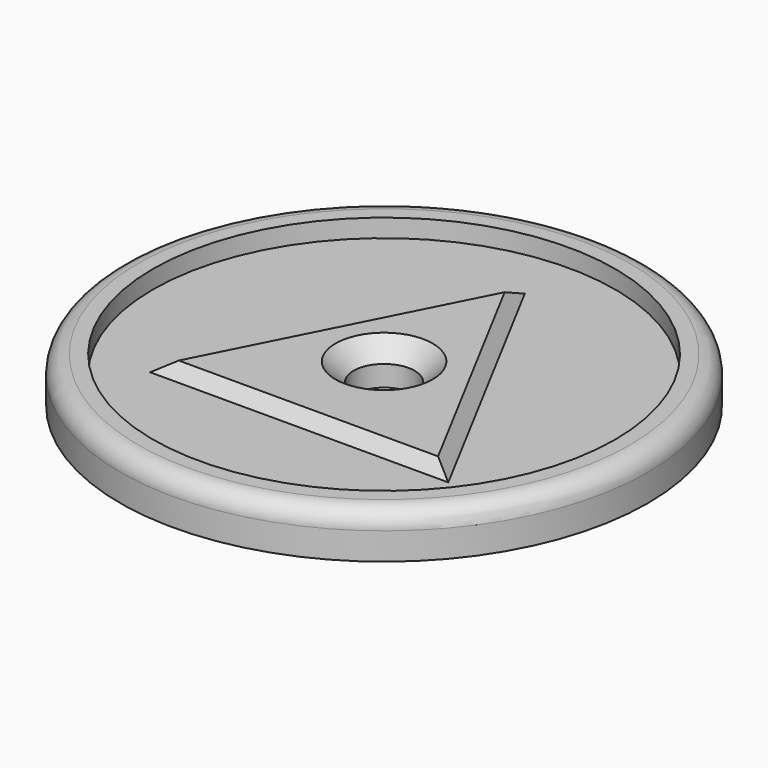
from build123d import *

# Parameters (mm, degrees)
F0_R         = 74.0650481318
F0_R_2       = 64.8450067866
F1_DEPTH     = 12.7
F2_DEPTH     = 7.62
F0_R_3       = 8.5707717009
F3_DEPTH     = 10.922
F4_R         = 5.08
F5_T4_DEPTH  = 123.6076762244
F5_T11_DEPTH = 122.6061545132
F5_T18_DEPTH = 115.6407516409


# Not quite as in the source:
# - a fillet or chamfer that OpenCascade refuses, or shapes differently, is made with other operations: its cross-section is extruded or revolved along the edge and cut away or added


with BuildPart() as f1:
    # F0 (on Top) → F1 (new body)
    with BuildSketch(Plane.XY):
        Circle(F0_R)
        Circle(F0_R_2, mode=Mode.SUBTRACT)
    extrude(amount=F1_DEPTH)

    # F0 (on Top) → F2 (join)
    with BuildSketch(Plane.XY):
        Circle(F0_R_2)
        Polygon((45.8412840962, -32.8662097454), (-43.6711683869, -32.8662097454), (0, 53.1617254019), align=None, mode=Mode.SUBTRACT)
    extrude(amount=F2_DEPTH)

    # F0 (on Top) → F3 (join)
    with BuildSketch(Plane.XY):
        Polygon((0, 53.1617254019), (-43.6711683869, -32.8662097454), (45.8412840962, -32.8662097454), align=None)
        Circle(F0_R_3, mode=Mode.SUBTRACT)
    extrude(amount=F3_DEPTH)

    # F4
    f4_edges = [f1.edges().sort_by_distance(p)[0] for p in [
        (-74.065048, 0, 12.7),
    ]]
    fillet(f4_edges, radius=F4_R)

    # F5: chamfer of 5.08 on 4 edges, made by hand


with BuildPart() as f5_tool2:
    # F5_s3 → F5_t4 (new body)
    with BuildSketch(Plane(origin=(29.9216472697, -56.1523871237, 0), x_dir=(0, 0, 1), z_dir=(-0.4702664859, 0.8825244655, 0))):
        Polygon((10.922, 19.9201777866), (5.842, 25.0001777866), (10.922, 25.0001777866), align=None)
    extrude(amount=F5_T4_DEPTH)

    split(bisect_by=Plane.XY.offset(7.62), keep=Keep.TOP)

    split(bisect_by=Plane(origin=(-21.4574493748, 10.8926464781, 0), x_dir=(0, 0, 1), z_dir=(0.8916858157, -0.4526548422, 0)), keep=Keep.TOP)

    split(bisect_by=Plane.XZ.offset(32.8662097454), keep=Keep.BOTTOM)


with BuildPart() as f1_1:
    add(f1.part)

    # F5_t1: cut F5_tool2
    add(f5_tool2.part, mode=Mode.SUBTRACT)


with BuildPart() as f5_tool9:
    # F5_s10 → F5_t11 (new body)
    with BuildSketch(Plane(origin=(27.3709999402, 53.9181957971, 0), x_dir=(0, 0, 1), z_dir=(-0.4526548422, -0.8916858157, 0))):
        Polygon((10.922, 18.9839124202), (5.842, 24.0639124202), (10.922, 24.0639124202), align=None)
    extrude(amount=F5_T11_DEPTH)

    split(bisect_by=Plane.XY.offset(7.62), keep=Keep.TOP)

    split(bisect_by=Plane(origin=(22.0632685396, 11.7567457534, 0), x_dir=(0, 0, 1), z_dir=(-0.8825244655, -0.4702664859, 0)), keep=Keep.TOP)

    split(bisect_by=Plane.XZ.offset(32.8662097454), keep=Keep.BOTTOM)


with BuildPart() as f1_2:
    add(f1_1.part)

    # F5_t8: cut F5_tool9
    add(f5_tool9.part, mode=Mode.SUBTRACT)


with BuildPart() as f5_tool16:
    # F5_s17 → F5_t18 (new body)
    with BuildSketch(Plane.YZ.offset(-56.7353179658)):
        Polygon((-27.7862097454, 10.922), (-32.8662097454, 5.842), (-32.8662097454, 10.922), align=None)
    extrude(amount=F5_T18_DEPTH)

    split(bisect_by=Plane.XY.offset(7.62), keep=Keep.TOP)

    split(bisect_by=Plane(origin=(22.0632685396, 11.7567457534, 0), x_dir=(0, 0, 1), z_dir=(-0.8825244655, -0.4702664859, 0)), keep=Keep.TOP)

    split(bisect_by=Plane(origin=(-21.4574493748, 10.8926464781, 0), x_dir=(0, 0, 1), z_dir=(0.8916858157, -0.4526548422, 0)), keep=Keep.TOP)


with BuildPart() as f1_3:
    add(f1_2.part)

    # F5_t15: cut F5_tool16
    add(f5_tool16.part, mode=Mode.SUBTRACT)

    # F5_s22 → F5_t23 (revolve, cut)
    with BuildSketch(Plane.XZ):
        Polygon((8.5707717009, 5.842), (13.6507717009, 10.922), (8.5707717009, 10.922), align=None)
    revolve(axis=Axis((0, 0, 10.922), (0, 0, 1)), mode=Mode.SUBTRACT)


solid = f1_3.part
